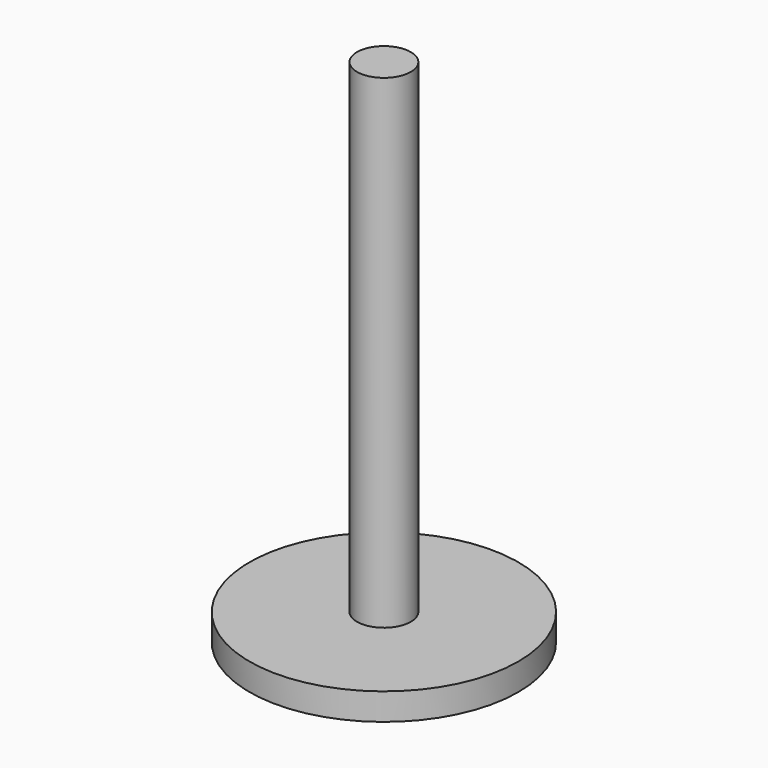
from build123d import *

# Parameters (mm, degrees)
F0_R     = 25
F1_DEPTH = 5
F2_R     = 5
F3_DEPTH = 90


# Not quite as in the source:
# - the program builds the solid bodies; features that only make, move or delete a surface that nothing else refers to are left out


with BuildPart() as f1:
    # F0 (on Top) → F1 (new body)
    with BuildSketch(Plane.XY):
        Circle(F0_R)
    extrude(amount=F1_DEPTH)

    # F2 (on face) → F3 (join)
    with BuildSketch(Plane.XY.offset(5)):
        Circle(F2_R)
    extrude(amount=F3_DEPTH)


solid = f1.part
